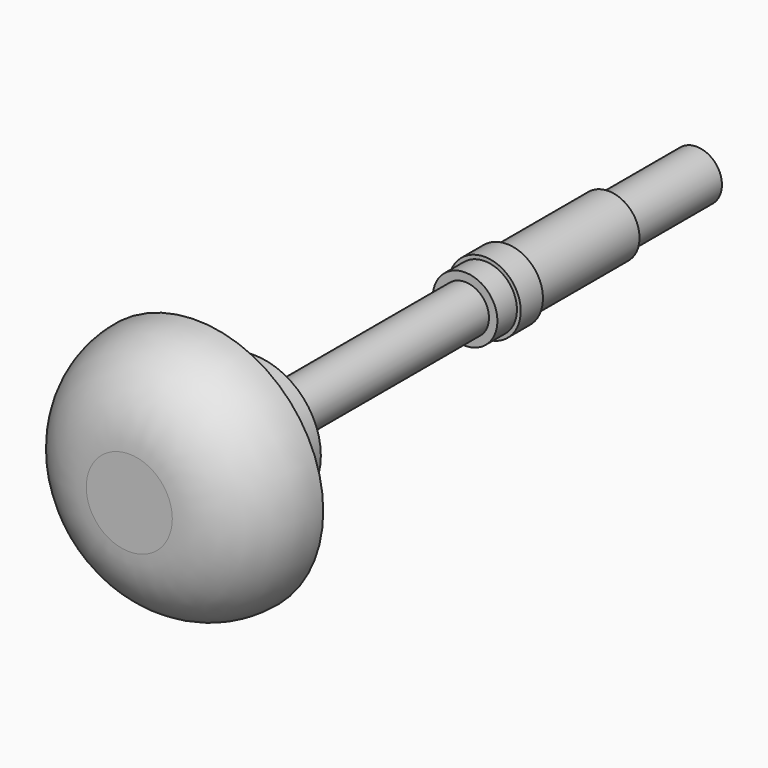
from build123d import *

# Parameters (mm, degrees)
F0_R      = 27.9630212455
F1_DEPTH  = 30
F2_R      = 52.9615929448
F2_R_2    = 27.9630212455
F3_DEPTH  = 35
F4_R      = 34.99999
F5_R      = 9.9870725783
F6_DEPTH  = 110.2
F7_R      = 13.4976595802
F7_R_2    = 9.9870725783
F8_DEPTH  = 10.2
F9_R      = 15.0753999454
F9_R_2    = 13.4976595802
F10_DEPTH = 11.6
F11_R     = 12.993046765
F12_DEPTH = 53
F13_R     = 10.5964364109
F14_DEPTH = 46


# Not quite as in the source:
# - a fillet or chamfer is up to 0.001 mm smaller than in the source, because OpenCascade refuses the exact size


with BuildPart() as f1:
    # F0 (on Front) → F1 (new body)
    with BuildSketch(Plane.XZ):
        with Locations((-0.0335160657, 0.0100570778)):
            Circle(F0_R)
    extrude(amount=F1_DEPTH)

    # F2 (on face) → F3 (join)
    with BuildSketch(Plane.XZ.offset(30)):
        with Locations((-0.0335160657, 0.0100570778)):
            Circle(F2_R)
        with Locations((-0.0335160657, 0.0100570778)):
            Circle(F2_R_2, mode=Mode.SUBTRACT)
        with Locations((-0.0335160657, 0.0100570778)):
            Circle(F2_R_2)
    extrude(amount=F3_DEPTH)

    # F4 (radius 35 in the source; OpenCascade refuses exactly that, so slightly less here)
    f4_edges = [f1.edges().sort_by_distance(p)[0] for p in [
        (-52.995109, -65, 0.010057),
    ]]
    fillet(f4_edges, radius=F4_R)

    # F5 (on face) → F6 (join)
    with BuildSketch(Plane(origin=(0, 0, 0), x_dir=(-1, 0, 0), z_dir=(0, 1, 0))):
        with Locations((0.0335160657, 0.0100570778)):
            Circle(F5_R)
    extrude(amount=F6_DEPTH)

    # F7 (on face) → F8 (join)
    with BuildSketch(Plane(origin=(0, 110.2, 0), x_dir=(-1, 0, 0), z_dir=(0, 1, 0))):
        with Locations((0.0335160657, 0.0100570778)):
            Circle(F7_R)
        with Locations((0.0335160657, 0.0100570778)):
            Circle(F7_R_2, mode=Mode.SUBTRACT)
        with Locations((0.0335160657, 0.0100570778)):
            Circle(F7_R_2)
    extrude(amount=F8_DEPTH)

    # F9 (on face) → F10 (join)
    with BuildSketch(Plane(origin=(0, 120.4, 0), x_dir=(-1, 0, 0), z_dir=(0, 1, 0))):
        with Locations((0.0335160657, 0.0100570778)):
            Circle(F9_R)
        with Locations((0.0335160657, 0.0100570778)):
            Circle(F9_R_2, mode=Mode.SUBTRACT)
        with Locations((0.0335160657, 0.0100570778)):
            Circle(F9_R_2)
    extrude(amount=F10_DEPTH)

    # F11 (on face) → F12 (join)
    with BuildSketch(Plane(origin=(0, 132, 0), x_dir=(-1, 0, 0), z_dir=(0, 1, 0))):
        with Locations((0.0335160657, 0.0100570778)):
            Circle(F11_R)
    extrude(amount=F12_DEPTH)

    # F13 (on face) → F14 (join)
    with BuildSketch(Plane(origin=(0, 185, 0), x_dir=(-1, 0, 0), z_dir=(0, 1, 0))):
        with Locations((0.0335160657, 0.0100570778)):
            Circle(F13_R)
    extrude(amount=F14_DEPTH)


solid = f1.part
